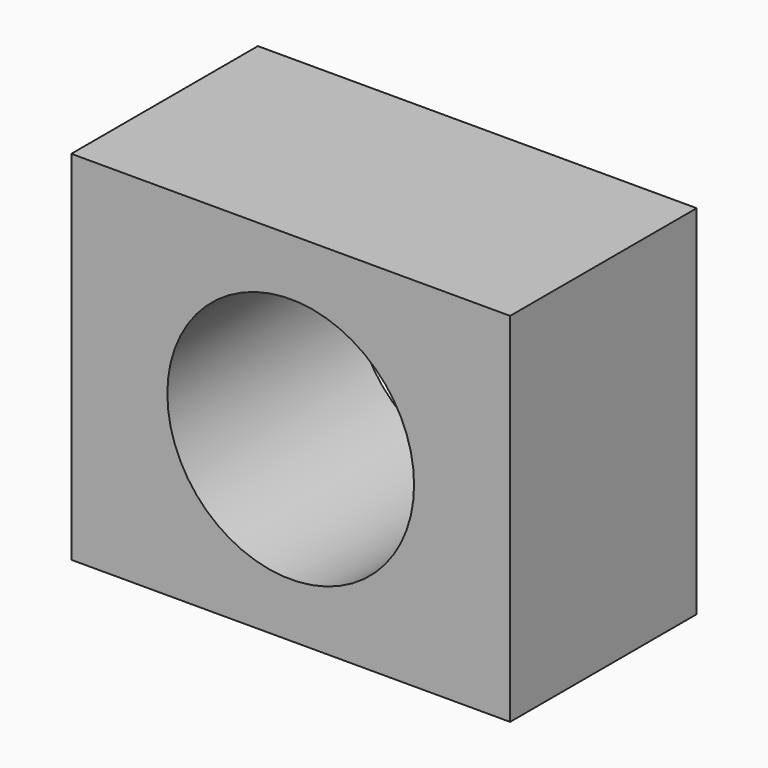
from build123d import *

# Parameters (mm, degrees)
F0_W     = 47.7912109345
F0_H     = 38.9310382307
F0_R     = 13.4352343475
F1_DEPTH = 25.4


# Not quite as in the source:
# - the program builds the solid bodies; features that only make, move or delete a surface that nothing else refers to are left out


with BuildPart() as f1:
    # F0 (on Front) → F1 (new body)
    with BuildSketch(Plane.XZ):
        with Locations((-41.750186123, 37.8570798784)):
            Rectangle(F0_W, F0_H)
        with Locations((-41.7501851916, 37.7228334546)):
            Circle(F0_R, mode=Mode.SUBTRACT)
    extrude(amount=F1_DEPTH)


solid = f1.part
